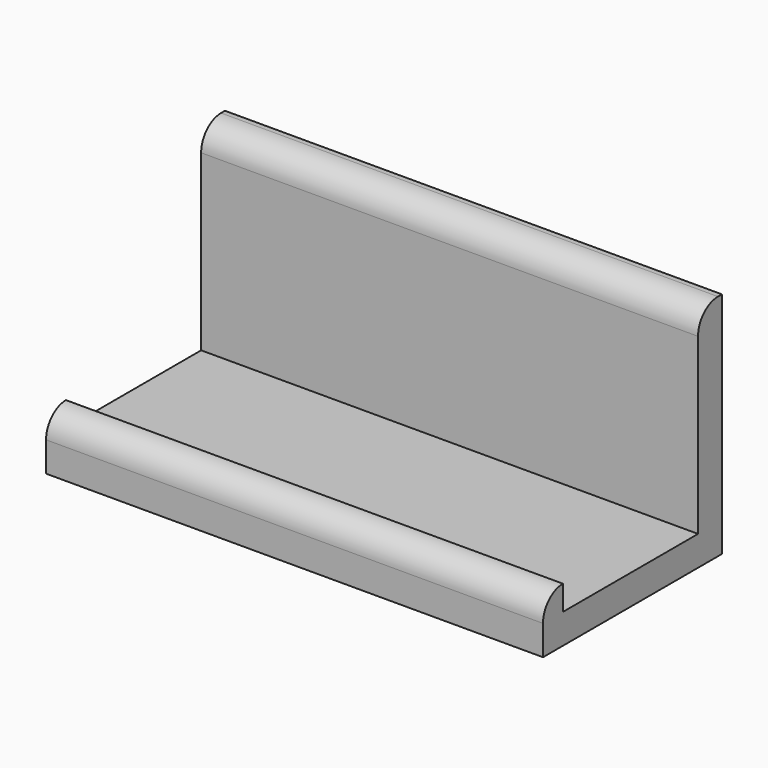
from build123d import *

# Parameters (mm, degrees)
F0_W     = 100
F0_H     = 45
F1_DEPTH = 6
F2_W     = 100
F2_H     = 5
F3_DEPTH = 5
F4_W     = 100
F4_H     = 6
F5_DEPTH = 40
F6_R     = 4.99999
F7_R     = 5


# Not quite as in the source:
# - a fillet or chamfer is up to 0.001 mm smaller than in the source, because OpenCascade refuses the exact size


with BuildPart() as f1:
    # F0 (on Top) → F1 (new body)
    with BuildSketch(Plane.XY):
        Rectangle(F0_W, F0_H)
    extrude(amount=F1_DEPTH)

    # F2 (on face) → F3 (join)
    with BuildSketch(Plane.XY.offset(6)):
        with Locations((0, -20)):
            Rectangle(F2_W, F2_H)
    extrude(amount=F3_DEPTH)

    # F4 (on face) → F5 (join)
    with BuildSketch(Plane.XY.offset(6)):
        with Locations((0, 19.5)):
            Rectangle(F4_W, F4_H)
    extrude(amount=F5_DEPTH)

    # F6 (radius 5 in the source; OpenCascade refuses exactly that, so slightly less here)
    f6_edges = [f1.edges().sort_by_distance(p)[0] for p in [
        (0, -22.5, 11),
    ]]
    fillet(f6_edges, radius=F6_R)

    # F7
    f7_edges = [f1.edges().sort_by_distance(p)[0] for p in [
        (0, 16.5, 46),
    ]]
    fillet(f7_edges, radius=F7_R)


solid = f1.part
